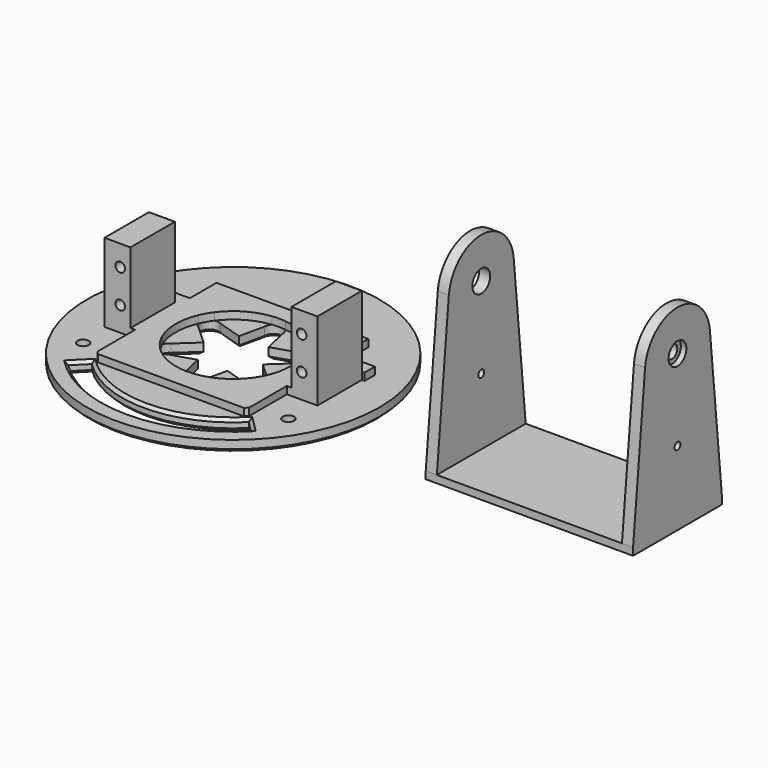
from build123d import *

# Parameters (mm, degrees)
F0_R      = 39.5
F0_R_2    = 1.5340881109
F1_DEPTH  = 3
F2_W      = 8.25
F2_H      = 15
F3_DEPTH  = 2
F4_W      = 7
F4_H      = 20.2
F4_R      = 1.3
F5_DEPTH  = 7.5
F6_W      = 56
F6_H      = 30
F7_DEPTH  = 2
F8_R      = 3
F8_R_2    = 1
F9_DEPTH  = 3
F13_DEPTH = 1.5
F14_R     = 3.8
F14_R_2   = 1.8
F15_DEPTH = 1.8
F16_SIZE  = 0.8
F18_DEPTH = 25
F19_SIZE  = 0.8


with BuildPart() as f1:
    # F0 (on Top) → F1 (new body)
    with BuildSketch(Plane.XY):
        Circle(F0_R)
        with Locations((-27.7128129211, -16)):
            Circle(F0_R_2, mode=Mode.SUBTRACT)
        with Locations((27.7128129211, -16)):
            Circle(F0_R_2, mode=Mode.SUBTRACT)
        with BuildLine():
            ThreePointArc((-2.5, 13.6782032303), (0, 16.1782032303), (2.5, 13.6782032303))
            Line((2.5, 13.6782032303), (4, 6.9282032303))
            Line((4, 6.9282032303), (10.5956714755, 9.0041651246))
            ThreePointArc((10.5956714755, 9.0041651246), (14.010734985, 8.0891016151), (13.0956714755, 4.6740381057))
            Line((13.0956714755, 4.6740381057), (8, 0))
            Line((8, 0), (13.0956714755, -4.6740381057))
            ThreePointArc((13.0956714755, -4.6740381057), (14.010734985, -8.0891016151), (10.5956714755, -9.0041651246))
            Line((10.5956714755, -9.0041651246), (4, -6.9282032303))
            Line((4, -6.9282032303), (2.5, -13.6782032303))
            ThreePointArc((2.5, -13.6782032303), (0, -16.1782032303), (-2.5, -13.6782032303))
            Line((-2.5, -13.6782032303), (-4, -6.9282032303))
            Line((-4, -6.9282032303), (-10.5956714755, -9.0041651246))
            ThreePointArc((-10.5956714755, -9.0041651246), (-14.010734985, -8.0891016151), (-13.0956714755, -4.6740381057))
            Line((-13.0956714755, -4.6740381057), (-8, 0))
            Line((-8, 0), (-13.0956714755, 4.6740381057))
            ThreePointArc((-13.0956714755, 4.6740381057), (-14.010734985, 8.0891016151), (-10.5956714755, 9.0041651246))
            Line((-10.5956714755, 9.0041651246), (-4, 6.9282032303))
            Line((-4, 6.9282032303), (-2.5, 13.6782032303))
        make_face(mode=Mode.SUBTRACT)
        with Locations((0, 32)):
            Circle(F0_R_2, mode=Mode.SUBTRACT)
    extrude(amount=F1_DEPTH)

    # F2 (on face) → F3 (join)
    with BuildSketch(Plane.XY.offset(3)):
        Polygon((-20.5, -21), (20.5, -21), (20.5, -7.5), (20.5, 7.5), (20.5, 11), (20.5, 20), (-20.5, 20), (-20.5, 11), (-20.5, 7.5), (-20.5, -7.5), align=None)
        with BuildLine():
            ThreePointArc((14.240270178, 6.120841875), (15.1818014043, 3.124564949), (15.5, 0))
            ThreePointArc((15.5, 0), (15.1818014043, -3.124564949), (14.240270178, -6.120841875))
            ThreePointArc((14.240270178, -6.120841875), (14.010734985, -8.0891016151), (12.4209396453, -9.2720147934))
            ThreePointArc((12.4209396453, -9.2720147934), (7.75, -13.4233937587), (1.8193305327, -15.3928566684))
            ThreePointArc((1.8193305327, -15.3928566684), (0, -16.1782032303), (-1.8193305327, -15.3928566684))
            ThreePointArc((-1.8193305327, -15.3928566684), (-7.75, -13.4233937587), (-12.4209396453, -9.2720147934))
            ThreePointArc((-12.4209396453, -9.2720147934), (-14.010734985, -8.0891016151), (-14.240270178, -6.120841875))
            ThreePointArc((-14.240270178, -6.120841875), (-15.5, 0), (-14.240270178, 6.120841875))
            ThreePointArc((-14.240270178, 6.120841875), (-14.010734985, 8.0891016151), (-12.4209396453, 9.2720147934))
            ThreePointArc((-12.4209396453, 9.2720147934), (-7.75, 13.4233937587), (-1.8193305327, 15.3928566684))
            ThreePointArc((-1.8193305327, 15.3928566684), (0, 16.1782032303), (1.8193305327, 15.3928566684))
            ThreePointArc((1.8193305327, 15.3928566684), (7.75, 13.4233937587), (12.4209396453, 9.2720147934))
            ThreePointArc((12.4209396453, 9.2720147934), (14.010734985, 8.0891016151), (14.240270178, 6.120841875))
        make_face(mode=Mode.SUBTRACT)
        with Locations((24.625, 0)):
            Rectangle(F2_W, F2_H)
        with Locations((-24.625, 0)):
            Rectangle(F2_W, F2_H)
        Polygon((20.5, 11), (20.5, 7.5), (28.75, 7.5), (29.5, 7.5), (29.5, 11), align=None)
        Polygon((-28.75, 7.5), (-20.5, 7.5), (-20.5, 11), (-29.5, 11), (-29.5, 7.5), align=None)
        with BuildLine():
            ThreePointArc((12.4209396453, 9.2720147934), (13.4233937587, 7.75), (14.240270178, 6.120841875))
            ThreePointArc((14.240270178, 6.120841875), (14.010734985, 8.0891016151), (12.4209396453, 9.2720147934))
        make_face()
        with BuildLine():
            ThreePointArc((12.4209396453, -9.2720147934), (14.010734985, -8.0891016151), (14.240270178, -6.120841875))
            ThreePointArc((14.240270178, -6.120841875), (13.4233937587, -7.75), (12.4209396453, -9.2720147934))
        make_face()
        with BuildLine():
            ThreePointArc((-1.8193305327, 15.3928566684), (0, 15.5), (1.8193305327, 15.3928566684))
            ThreePointArc((1.8193305327, 15.3928566684), (0, 16.1782032303), (-1.8193305327, 15.3928566684))
        make_face()
        with BuildLine():
            ThreePointArc((-1.8193305327, -15.3928566684), (0, -16.1782032303), (1.8193305327, -15.3928566684))
            ThreePointArc((1.8193305327, -15.3928566684), (0, -15.5), (-1.8193305327, -15.3928566684))
        make_face()
        with BuildLine():
            ThreePointArc((-14.240270178, 6.120841875), (-13.4233937587, 7.75), (-12.4209396453, 9.2720147934))
            ThreePointArc((-12.4209396453, 9.2720147934), (-14.010734985, 8.0891016151), (-14.240270178, 6.120841875))
        make_face()
        with BuildLine():
            ThreePointArc((-14.240270178, -6.120841875), (-14.010734985, -8.0891016151), (-12.4209396453, -9.2720147934))
            ThreePointArc((-12.4209396453, -9.2720147934), (-13.4233937587, -7.75), (-14.240270178, -6.120841875))
        make_face()
    extrude(amount=F3_DEPTH)

    # F4 (on Front) → F5 (join, symmetric)
    with BuildSketch(Plane.XZ):
        with Locations((25.25, 14.1)):
            Rectangle(F4_W, F4_H)
        with Locations((24.5, 9.6)):
            Circle(F4_R, mode=Mode.SUBTRACT)
        with Locations((24.5, 18.6)):
            Circle(F4_R, mode=Mode.SUBTRACT)
        with Locations((-25.25, 14.1)):
            Rectangle(F4_W, F4_H)
        with Locations((-24.5, 9.6)):
            Circle(F4_R, mode=Mode.SUBTRACT)
        with Locations((-24.5, 18.6)):
            Circle(F4_R, mode=Mode.SUBTRACT)
    extrude(amount=F5_DEPTH, both=True)

    # F17 (on face) → F18 (cut)
    with BuildSketch(Plane.XY.offset(3)):
        with BuildLine():
            Line((-21.2132034356, -21.2132034356), (-24.7487373415, -24.7487373415))
            ThreePointArc((-24.7487373415, -24.7487373415), (0, -35), (24.7487373415, -24.7487373415))
            Line((24.7487373415, -24.7487373415), (21.2132034356, -21.2132034356))
            ThreePointArc((21.2132034356, -21.2132034356), (0, -30), (-21.2132034356, -21.2132034356))
        make_face()
    extrude(amount=-F18_DEPTH, mode=Mode.SUBTRACT)

    # F19 (call 1 of 9: OpenCascade refuses the feature's edges together)
    f19_edges = [f1.edges().sort_by_distance(p)[0] for p in [
        (-20.5, -21, 4),
    ]]
    chamfer(f19_edges, length=F19_SIZE)

    # F19#2 (call 2 of 9)
    f19_2_edges = [f1.edges().sort_by_distance(p)[0] for p in [
        (20.5, -21, 4),
    ]]
    chamfer(f19_2_edges, length=F19_SIZE)

    # F19#3 (call 3 of 9)
    f19_3_edges = [f1.edges().sort_by_distance(p)[0] for p in [
        (0, -30, 3),
        (-22.98097, -22.98097, 3),
        (0, -35, 3),
        (22.98097, -22.98097, 3),
    ]]
    chamfer(f19_3_edges, length=F19_SIZE)

    # F19#4 (call 4 of 9)
    f19_4_edges = [f1.edges().sort_by_distance(p)[0] for p in [
        (0, -30, 0),
        (-22.98097, -22.98097, 0),
        (0, -35, 0),
        (22.98097, -22.98097, 0),
    ]]
    chamfer(f19_4_edges, length=F19_SIZE)

    # F19#5 (call 5 of 9)
    f19_5_edges = [f1.edges().sort_by_distance(p)[0] for p in [
        (-39.5, 0, 0),
    ]]
    chamfer(f19_5_edges, length=F19_SIZE)

    # F19#6 (call 6 of 9)
    f19_6_edges = [f1.edges().sort_by_distance(p)[0] for p in [
        (-29.246901, -16, 0),
    ]]
    chamfer(f19_6_edges, length=F19_SIZE)

    # F19#7 (call 7 of 9)
    f19_7_edges = [f1.edges().sort_by_distance(p)[0] for p in [
        (26.178725, -16, 0),
    ]]
    chamfer(f19_7_edges, length=F19_SIZE)

    # F19#8 (call 8 of 9)
    f19_8_edges = [f1.edges().sort_by_distance(p)[0] for p in [
        (-14.010735, -8.089102, 0),
        (-7.297836, -7.966184, 0),
        (-10.547836, -2.337019, 0),
        (-3.25, -10.303203, 0),
        (-10.547836, 2.337019, 0),
        (0, -16.178203, 0),
        (-14.010735, 8.089102, 0),
        (3.25, -10.303203, 0),
        (-7.297836, 7.966184, 0),
        (7.297836, -7.966184, 0),
        (-3.25, 10.303203, 0),
        (14.010735, -8.089102, 0),
        (0, 16.178203, 0),
        (10.547836, -2.337019, 0),
        (3.25, 10.303203, 0),
        (10.547836, 2.337019, 0),
        (7.297836, 7.966184, 0),
        (14.010735, 8.089102, 0),
    ]]
    chamfer(f19_8_edges, length=F19_SIZE)

    # F19#9 (call 9 of 9)
    f19_9_edges = [f1.edges().sort_by_distance(p)[0] for p in [
        (-1.534088, 32, 0),
    ]]
    chamfer(f19_9_edges, length=F19_SIZE)


with BuildPart() as f7:
    # F6 (on Top) → F7 (new body)
    with BuildSketch(Plane.XY):
        with Locations((92.0131745475, 0)):
            Rectangle(F6_W, F6_H)
    extrude(amount=F7_DEPTH)


with BuildPart() as f9:
    # F8 (on face) → F9 (new body)
    with BuildSketch(Plane.YZ.offset(120.0131745475)):
        with BuildLine():
            ThreePointArc((-10.9468467659, 43.0800675372), (-0.5406873291, 31.0132963446), (11, 42))
            ThreePointArc((11, 42), (10.9867036554, 42.5406873291), (10.9468467659, 43.0800675372))
            ThreePointArc((10.9468467659, 43.0800675372), (0, 53), (-10.9468467659, 43.0800675372))
        make_face()
        with Locations((0, 42)):
            Circle(F8_R, mode=Mode.SUBTRACT)
        with BuildLine():
            ThreePointArc((10.9468467659, 43.0800675372), (10.9867036554, 42.5406873291), (11, 42))
            ThreePointArc((11, 42), (-0.5406873291, 31.0132963446), (-10.9468467659, 43.0800675372))
            Line((-10.9468467659, 43.0800675372), (-15, 2))
            Line((-15, 2), (0, 2))
            Line((0, 2), (15, 2))
            Line((15, 2), (10.9468467659, 43.0800675372))
        make_face()
        with Locations((0, 20)):
            Circle(F8_R_2, mode=Mode.SUBTRACT)
    extrude(amount=-F9_DEPTH)


with BuildPart() as f10_1:
    # F10: copy of F9
    add(f9.part.moved(Location((-53, 0, 0))))


with BuildPart() as f7_1:
    add(f7.part)

    # F11: union F9, F10_1
    add(f9.part)
    add(f10_1.part)

    # F12 (on face) → F13 (cut)
    with BuildSketch(Plane(origin=(117.0131745475, 0, 0), x_dir=(0, -1, 0), z_dir=(-1, 0, 0))):
        with BuildLine():
            ThreePointArc((6.9317780118, 41.0250879041), (6.9829236743, 41.5113519072), (7, 42))
            ThreePointArc((7, 42), (-0.4886480928, 48.9829236743), (-6.9317780118, 41.0250879041))
            ThreePointArc((-6.9317780118, 41.0250879041), (0, 35), (6.9317780118, 41.0250879041))
        make_face()
        with BuildLine():
            ThreePointArc((6.9317780118, 41.0250879041), (0, 35), (-6.9317780118, 41.0250879041))
            Line((-6.9317780118, 41.0250879041), (-6, 34.4))
            Line((-6, 34.4), (0, 34.4))
            Line((0, 34.4), (6, 34.4))
            Line((6, 34.4), (6.9317780118, 41.0250879041))
        make_face()
    extrude(amount=-F13_DEPTH, mode=Mode.SUBTRACT)

    # F14 (on face) → F15 (join)
    with BuildSketch(Plane(origin=(118.5131745475, 0, 0), x_dir=(0, -1, 0), z_dir=(-1, 0, 0))):
        with Locations((0, 42)):
            Circle(F14_R)
        with Locations((0, 42)):
            Circle(F14_R_2, mode=Mode.SUBTRACT)
    extrude(amount=F15_DEPTH)

    # F16
    f16_edges = [f7_1.edges().sort_by_distance(p)[0] for p in [
        (118.513175, 0, 49),
        (116.713175, 3.8, 42),
    ]]
    chamfer(f16_edges, length=F16_SIZE)


solid = Compound([f1.part, f7_1.part])
